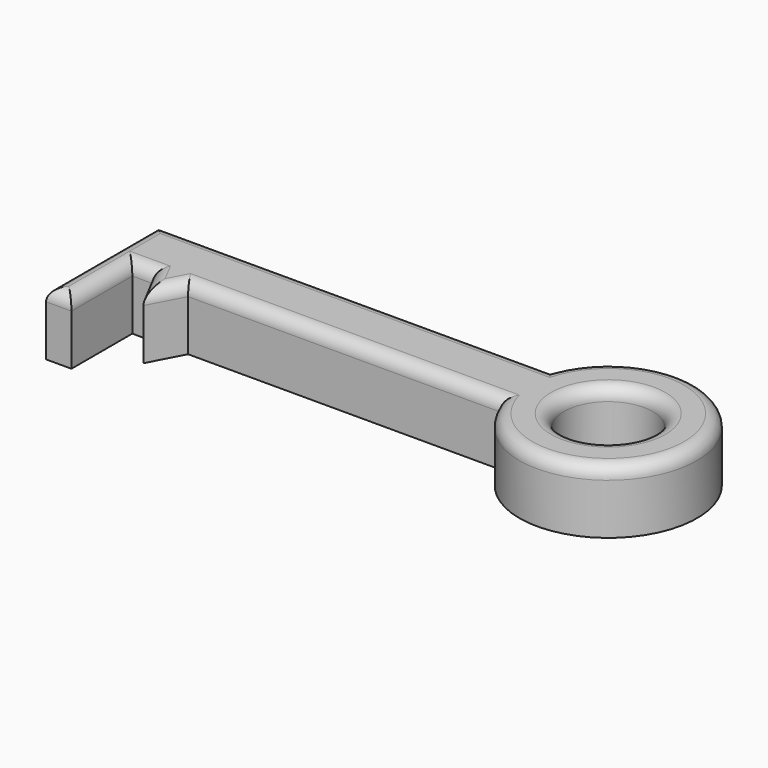
from build123d import *

# Parameters (mm, degrees)
F0_R     = 17.5
F0_W     = 8
F0_H     = 15
F1_DEPTH = 25
F2_R     = 4.99999


# Not quite as in the source:
# - a fillet or chamfer is up to 0.001 mm smaller than in the source, because OpenCascade refuses the exact size


with BuildPart() as f1:
    # F0 (on Top) → F1 (new body)
    with BuildSketch(Plane.XY):
        with BuildLine():
            Line((0, 3.9768594503), (-155, 3.9768594503))
            Line((-155, 3.9768594503), (-155, -21.0231405497))
            Line((-155, -21.0231405497), (-147, -21.0231405497))
            Line((-147, -21.0231405497), (-145, -21.0231405497))
            Line((-145, -21.0231405497), (-137, -21.0231405497))
            Line((-137, -21.0231405497), (-123, -21.0231405497))
            Line((-123, -21.0231405497), (0, -21.0231405497))
            ThreePointArc((0, -21.0231405497), (67.6917420766, -8.5231405497), (0, 3.9768594503))
        make_face()
        with Locations((32.6917420766, -8.5231405497)):
            Circle(F0_R, mode=Mode.SUBTRACT)
        with Locations((-151, -28.5231405497)):
            Rectangle(F0_W, F0_H)
        Polygon((-145, -21.0231405497), (-147, -21.0231405497), (-147, -36.0231405497), (-155, -36.0231405497), (-155, -51.0231405497), (-145, -51.0231405497), align=None)
        Polygon((-130, -34.2896397111), (-123, -21.0231405497), (-137, -21.0231405497), align=None)
    extrude(amount=F1_DEPTH)

    # F2 (radius 5 in the source; OpenCascade refuses exactly that, so slightly less here)
    f2_edges = [f1.edges().sort_by_distance(p)[0] for p in [
        (-77.5, 3.976859, 25),
        (-61.5, -21.023141, 25),
        (-133.5, -27.65639, 25),
        (-155, -23.523141, 25),
        (-145, -36.023141, 25),
        (67.691742, -8.523141, 25),
        (-150, -51.023141, 25),
        (-141, -21.023141, 25),
        (-126.5, -27.65639, 25),
        (15.191742, -8.523141, 25),
    ]]
    fillet(f2_edges, radius=F2_R)


solid = f1.part
